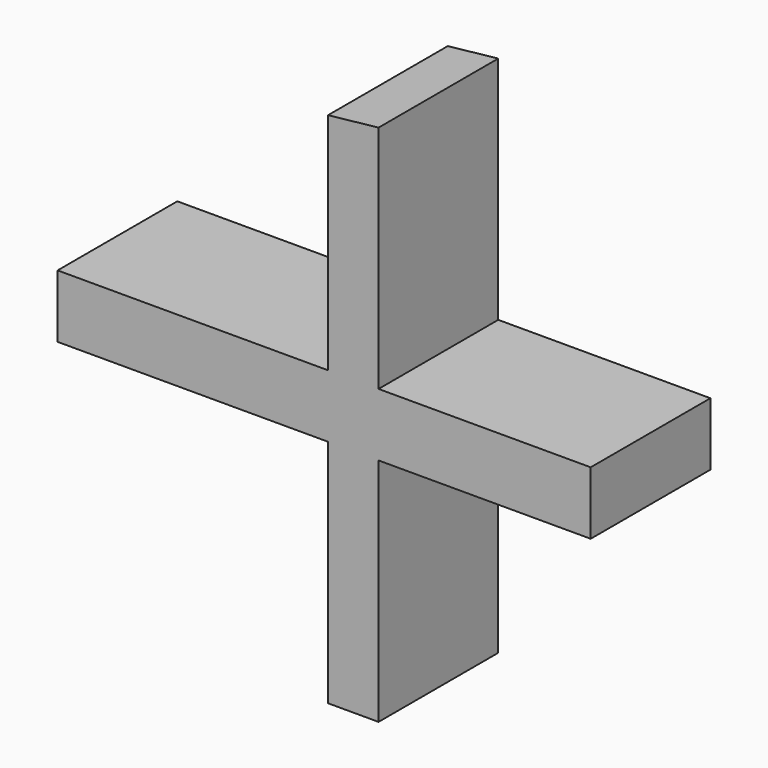
from build123d import *

# Parameters (mm, degrees)
F0_W     = 45.9087826312
F0_H     = 10.6835663319
F0_W_2   = 8.5728019476
F0_W_3   = 36.0127463937
F1_DEPTH = 25.4
F0_H_2   = 39.0786156058
F2_DEPTH = 25.4


# Not quite as in the source:
# - a feature names something its author has since deleted; it is built from what else it names


with BuildPart() as f1:
    # F0 (on Front) → F1 (new body)
    with BuildSketch(Plane.XZ):
        with Locations((-31.5271932632, 44.4203987718)):
            Rectangle(F0_W, F0_H)
        with Locations((-4.2864009738, 44.4203987718)):
            Rectangle(F0_W_2, F0_H)
        with Locations((18.0063731968, 44.4203987718)):
            Rectangle(F0_W_3, F0_H)
    extrude(amount=F1_DEPTH)

    # F0 (on Front) → F2 (join)
    with BuildSketch(Plane.XZ):
        with Locations((-4.2864009738, 19.5393078029)):
            Rectangle(F0_W_2, F0_H_2)
        with Locations((-4.2864009738, 44.4203987718)):
            Rectangle(F0_W_2, F0_H)
        Polygon((-8.5728019476, 87.886022841), (-8.5728019476, 49.7621819377), (0, 49.7621819377), (0, 88.8135335598), align=None)
    extrude(amount=F2_DEPTH)


solid = f1.part
